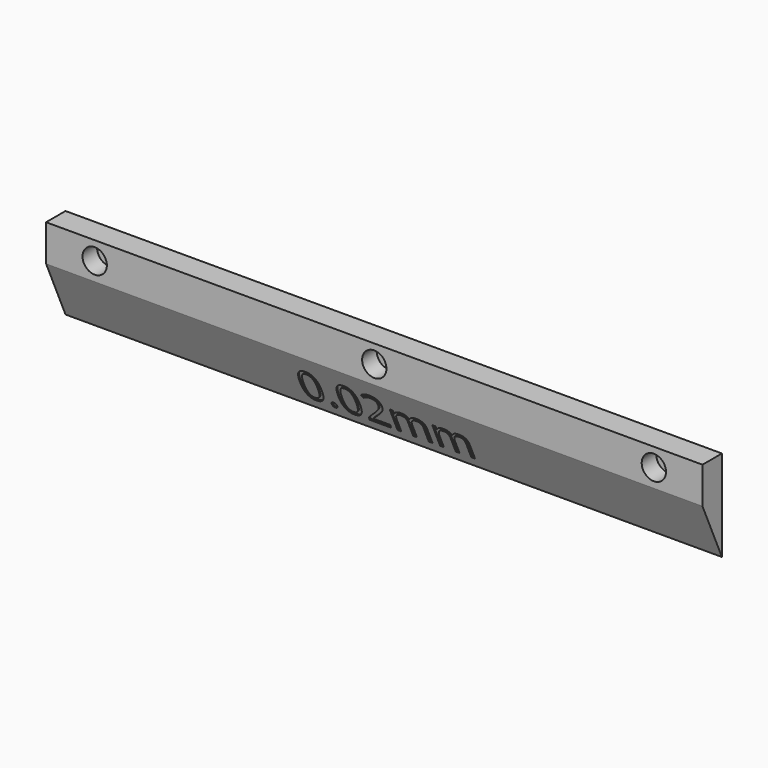
from build123d import *

# Parameters (mm, degrees)
F0_W         = 54
F0_H         = 7.5
F1_DEPTH     = 2
F3_DEPTH     = 54.001
F4_R         = 1
F5_DEPTH     = 1.5
F6_R         = 0.5
F7_DEPTH     = 0.501
F8_TEXT_SIZE = 3.7641675186
F9_DEPTH     = 0.1


# Not quite as in the source:
# - Text() gives the source's letters only with a copy of the font that has no kerning and outlines rounded to 1/6400 em; it was checked with that copy


with BuildPart() as f1:
    # F0 (on Front) → F1 (new body)
    with BuildSketch(Plane.XZ):
        with Locations((27, 3.75)):
            Rectangle(F0_W, F0_H)
    extrude(amount=F1_DEPTH)

    # F2 (on face) → F3 (cut, through all)
    with BuildSketch(Plane.YZ.offset(54)):
        Polygon((-2, 0), (0, 0), (-2, 4.4920735478), align=None)
    extrude(amount=-F3_DEPTH, mode=Mode.SUBTRACT)

    # F4 (on face) → F5 (cut)
    with BuildSketch(Plane.XZ.offset(2)):
        with Locations((4, 5.9970735478)):
            Circle(F4_R)
        with Locations((27, 5.9970735478)):
            Circle(F4_R)
        with Locations((50, 5.9970735478)):
            Circle(F4_R)
    extrude(amount=-F5_DEPTH, mode=Mode.SUBTRACT)

    # F6 (on face) → F7 (cut, through all)
    with BuildSketch(Plane.XZ.offset(0.5)):
        with Locations((4, 5.9970735478)):
            Circle(F6_R)
        with Locations((27, 5.9970735478)):
            Circle(F6_R)
        with Locations((50, 5.9970735478)):
            Circle(F6_R)
    extrude(amount=-F7_DEPTH, mode=Mode.SUBTRACT)

    # F8 (on face) → F9 (cut)
    with BuildSketch(Plane(origin=(0, 0, 0), x_dir=(1, 0, 0), z_dir=(0, -0.9135454576, -0.4067366431))):
        with Locations((19.8004414696, 0.8)):
            Text('0.02mm', F8_TEXT_SIZE, font='Open Sans', text_align=(TextAlign.LEFT, TextAlign.BOTTOM))
    extrude(amount=-F9_DEPTH, mode=Mode.SUBTRACT)


solid = f1.part
